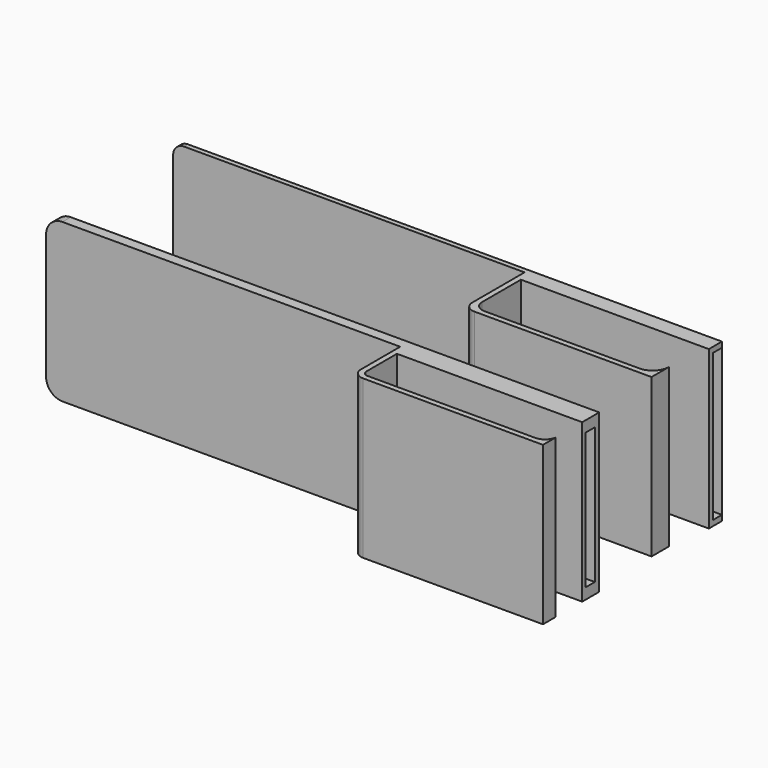
from build123d import *

# Parameters (mm, degrees)
F1_DEPTH  = 1.9
F0_W      = 35
F0_H      = 29
F2_DEPTH  = 12.9
F3_W      = 2.1
F3_H      = 25
F4_DEPTH  = 25
F5_R      = 2
F7_DEPTH  = 29
F9_DEPTH  = 29
F10_W     = 2
F10_H     = 27
F11_DEPTH = 25
F14_R     = 2
F15_SIZE  = 0.99999


# Not quite as in the source:
# - a fillet or chamfer is up to 0.001 mm smaller than in the source, because OpenCascade refuses the exact size


with BuildPart() as f1:
    # F0 (on Front) → F1 (new body)
    with BuildSketch(Plane.XZ):
        with BuildLine():
            Line((-97, 0), (-35, 0))
            Line((-35, 0), (-35, 29))
            Line((-35, 29), (-97, 29))
            ThreePointArc((-97, 29), (-99.1213203436, 28.1213203436), (-100, 26))
            Line((-100, 26), (-100, 3))
            ThreePointArc((-100, 3), (-99.1213203436, 0.8786796564), (-97, 0))
        make_face()
    extrude(amount=F1_DEPTH)

    # F0 (on Front) → F2 (join)
    with BuildSketch(Plane.XZ):
        with Locations((-17.5, 14.5)):
            Rectangle(F0_W, F0_H)
    extrude(amount=F2_DEPTH)

    # F3 (on face) → F4 (cut)
    with BuildSketch(Plane.YZ):
        with Locations((-2.05, 14.5)):
            Rectangle(F3_W, F3_H)
    extrude(amount=-F4_DEPTH, mode=Mode.SUBTRACT)

    # F5
    f5_edges = [f1.edges().sort_by_distance(p)[0] for p in [
        (-35, -12.9, 14.5),
    ]]
    fillet(f5_edges, radius=F5_R)

    # F6 (on face) → F7 (cut)
    with BuildSketch(Plane.XY.offset(29)):
        with BuildLine():
            Line((-34.0000018477, -3.9), (-34.0000018477, -10.9))
            ThreePointArc((-34.0000018477, -10.9), (-33.7071080877, -11.6071080877), (-33, -11.9000018477))
            Line((-33, -11.9000018477), (-2.4920476135, -11.9000018477))
            Line((-2.4920476135, -11.9000018477), (-2.0143143377, -11.9000018477))
            ThreePointArc((-2.0143143377, -11.9000018477), (-0.7060689283, -11.3136245624), (0, -10.0659022213))
            Line((0, -10.0659022213), (0, -9.1630909592))
            Line((0, -9.1630909592), (0, -3.9))
            Line((0, -3.9), (-34.0000018477, -3.9))
        make_face()
    extrude(amount=-F7_DEPTH, mode=Mode.SUBTRACT)


with BuildPart() as f9:
    # F8 (on Top) → F9 (new body)
    with BuildSketch(Plane.XY):
        with BuildLine():
            Line((0, 25.1590552804), (0, 29.1590552804))
            Line((0, 29.1590552804), (-100, 29.1590552804))
            Line((-100, 29.1590552804), (-100, 27.2590552804))
            Line((-100, 27.2590552804), (-35.5, 27.2590552804))
            Line((-35.5, 27.2590552804), (-35.5, 15.2590552804))
            ThreePointArc((-35.5, 15.2590552804), (-34.9142135624, 13.8448417181), (-33.5, 13.2590552804))
            Line((-33.5, 13.2590552804), (-1, 13.2590552804))
            Line((-1, 13.2590552804), (-1, 17.2590552804))
            ThreePointArc((-1, 17.2590552804), (-1.8786796564, 15.1377349369), (-4, 14.2590552804))
            Line((-4, 14.2590552804), (-32.5, 14.2590552804))
            ThreePointArc((-32.5, 14.2590552804), (-33.9142135624, 14.8448417181), (-34.5, 16.2590552804))
            Line((-34.5, 16.2590552804), (-34.5, 25.1590552804))
            Line((-34.5, 25.1590552804), (0, 25.1590552804))
        make_face()
    extrude(amount=F9_DEPTH)

    # F10 (on face) → F11 (cut)
    with BuildSketch(Plane.YZ):
        with Locations((27.1590552804, 14.5)):
            Rectangle(F10_W, F10_H)
    extrude(amount=-F11_DEPTH, mode=Mode.SUBTRACT)


with BuildPart() as f12_1:
    # F12: copy of F9
    add(f9.part.moved(Location((0, 30, 0))))


with BuildPart() as f9_1:
    add(f9.part)

    # F14
    f14_edges = [f9_1.edges().sort_by_distance(p)[0] for p in [
        (-100, 28.209055, 29),
        (-100, 28.209055, 0),
    ]]
    fillet(f14_edges, radius=F14_R)

    # F15 (size 1 in the source; OpenCascade refuses exactly that, so slightly less here)
    f15_edges = [f9_1.edges().sort_by_distance(p)[0] for p in [
        (-100, 29.159055, 14.5),
        (-99.414214, 29.159055, 0.585786),
        (-99.414214, 29.159055, 28.414214),
        (-49, 29.159055, 0),
        (-49, 29.159055, 29),
        (0, 29.159055, 14.5),
    ]]
    chamfer(f15_edges, length=F15_SIZE)


solid = Compound([f1.part, f9_1.part])
